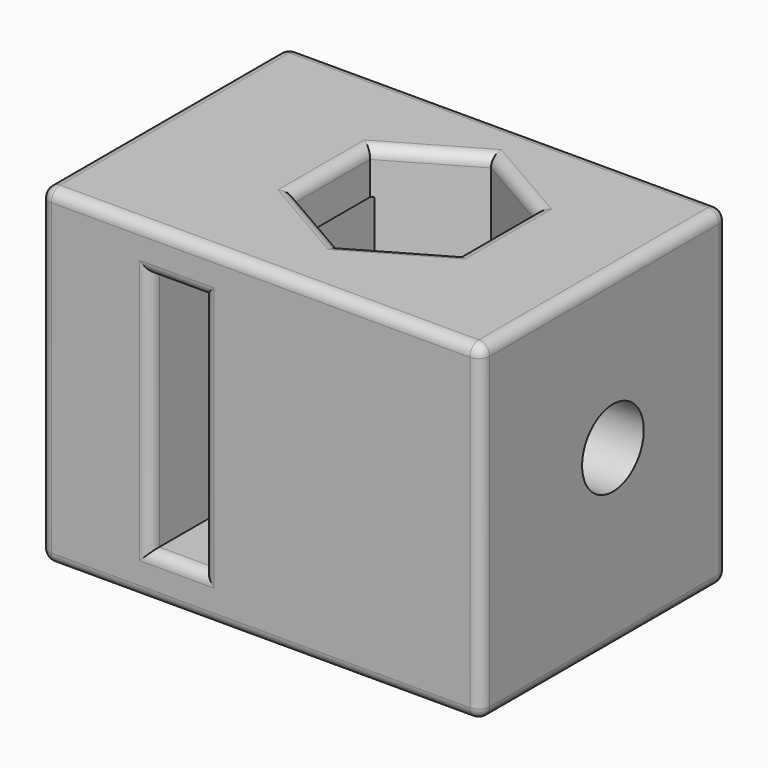
from build123d import *

# Parameters (mm, degrees)
F0_W          = 20
F0_H          = 14
F1_DEPTH      = 15
F2_W          = 2.39
F2_H          = 11
F3_DEPTH      = 14.001
F5_R          = 0.5
F4_R          = 1.75
F6_DEPTH      = 42
F6_DEPTH_BACK = 20.001


# Not quite as in the source:
# - an extrude ends at something that could not be found from the text; its depth is read off the source's solid


with BuildPart() as f1:
    # F0 (on Top) → F1 (new body)
    with BuildSketch(Plane.XY):
        with Locations((-1, -0.4900455125)):
            Rectangle(F0_W, F0_H)
        Polygon((3.75, -2.1650635095), (0, -4.3301270189), (-3.75, -2.1650635095), (-3.75, 2.1650635095), (0, 4.3301270189), (3.75, 2.1650635095), align=None, mode=Mode.SUBTRACT)
    extrude(amount=F1_DEPTH)

    # F2 (on face) → F3 (cut, through all)
    with BuildSketch(Plane.XZ.offset(7.4900455125)):
        with Locations((-4.805, 7.5)):
            Rectangle(F2_W, F2_H)
    extrude(amount=-F3_DEPTH, mode=Mode.SUBTRACT)

    # F5
    f5_edges = [f1.edges().sort_by_distance(p)[0] for p in [
        (-11, -7.490046, 7.5),
        (-1, -7.490046, 0),
        (-1, -7.490046, 15),
        (9, -7.490046, 7.5),
        (-3.61, -7.490046, 7.5),
        (-4.805, -7.490046, 2),
        (-6, -7.490046, 7.5),
        (-4.805, -7.490046, 13),
        (9, 6.509954, 7.5),
        (-1, 6.509954, 0),
        (-1, 6.509954, 15),
        (-11, 6.509954, 7.5),
        (-4.805, 6.509954, 13),
        (-6, 6.509954, 7.5),
        (-4.805, 6.509954, 2),
        (-3.61, 6.509954, 7.5),
        (9, -0.490046, 15),
        (-11, -0.490046, 15),
        (3.75, 0, 15),
        (1.875, -3.247595, 15),
        (-1.875, -3.247595, 15),
        (-3.75, 0, 15),
        (-1.875, 3.247595, 15),
        (1.875, 3.247595, 15),
        (9, -0.490046, 0),
        (-11, -0.490046, 0),
        (3.75, 0, 0),
        (1.875, -3.247595, 0),
        (-1.875, -3.247595, 0),
        (-3.75, 0, 0),
        (-1.875, 3.247595, 0),
        (1.875, 3.247595, 0),
    ]]
    fillet(f5_edges, radius=F5_R)

    # F4 (on face) → F6 (cut, two sides)
    with BuildSketch(Plane(origin=(-11, 0, 0), x_dir=(0, -1, 0), z_dir=(-1, 0, 0))) as f6_sk:
        with Locations((0, 8)):
            Circle(F4_R)
    extrude(amount=F6_DEPTH, mode=Mode.SUBTRACT)
    extrude(f6_sk.sketch, amount=-F6_DEPTH_BACK, mode=Mode.SUBTRACT)


solid = f1.part
